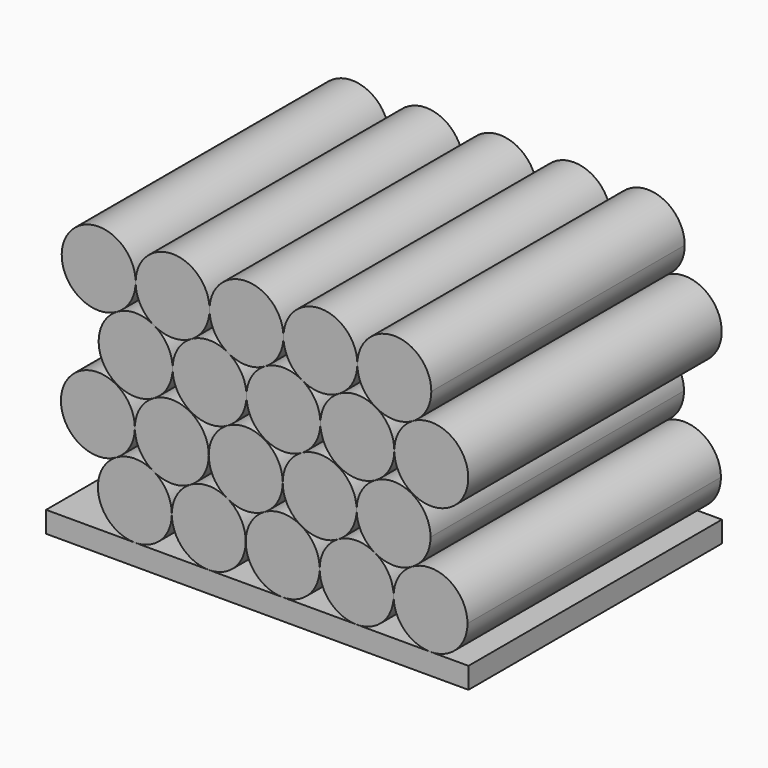
from build123d import *

# Parameters (mm, degrees)
F1_DEPTH = 76.2


# Not quite as in the source:
# - a feature names something its author has since deleted; it is built from what else it names


with BuildPart() as f1:
    # F0 (on Front) → F1 (new body)
    with BuildSketch(Plane.XZ):
        with BuildLine():
            ThreePointArc((-29.4477027383, -25.4555717693), (-23.1615234536, -22.851751054), (-20.5577027383, -16.5655717693))
            ThreePointArc((-20.5577027383, -16.5655717693), (-21.7487368667, -12.1205718246), (-25.0027026277, -8.8666059935))
            ThreePointArc((-25.0027026277, -8.8666059935), (-29.4477026803, -7.6755717693), (-33.8927027485, -8.8666059355))
            ThreePointArc((-33.8927027485, -8.8666059355), (-38.0347833325, -18.8664730859), (-29.4477027383, -25.4555717693))
        make_face()
    extrude(amount=F1_DEPTH)


with BuildPart() as f1b:
    # F0 (on Front) → F1, piece 2 (new body)
    with BuildSketch(Plane.XZ):
        with BuildLine():
            ThreePointArc((-16.1127027426, -8.8666059321), (-19.3666685792, -12.1205717714), (-20.5577027383, -16.5655717693))
            ThreePointArc((-20.5577027383, -16.5655717693), (-17.9538820218, -22.8517510553), (-11.6677027346, -25.4555717693))
            ThreePointArc((-11.6677027346, -25.4555717693), (-5.3815234523, -22.8517510527), (-2.7777027383, -16.5655717693))
            ThreePointArc((-2.7777027383, -16.5655717693), (-3.9687368512, -12.1205718515), (-7.2227025739, -8.8666060246))
            ThreePointArc((-7.2227025739, -8.8666060246), (-11.6677026458, -7.6755717693), (-16.1127027426, -8.8666059321))
        make_face()
    extrude(amount=F1_DEPTH)


with BuildPart() as f1c:
    # F0 (on Front) → F1, piece 3 (new body)
    with BuildSketch(Plane.XZ):
        with BuildLine():
            ThreePointArc((-29.4477027383, -1.16764009), (-28.256668546, -5.6126401453), (-25.0027026277, -8.8666059935))
            ThreePointArc((-25.0027026277, -8.8666059935), (-20.5577026769, -10.05764009), (-16.1127027426, -8.8666059321))
            ThreePointArc((-16.1127027426, -8.8666059321), (-12.8587368999, -5.6126400921), (-11.6677027383, -1.16764009))
            ThreePointArc((-11.6677027383, -1.16764009), (-16.0669411864, 6.5047233453), (-24.9107085164, 6.5837108049))
            ThreePointArc((-24.9107085164, 6.5837108049), (-28.2300661736, 3.323121462), (-29.4477027383, -1.16764009))
        make_face()
    extrude(amount=F1_DEPTH)


with BuildPart() as f1d:
    # F0 (on Front) → F1, piece 4 (new body)
    with BuildSketch(Plane.XZ):
        Polygon((-11.6677027346, -25.4555717693), (-29.4477027383, -25.4555717693), (-50.8, -25.4555717693), (-50.8, -30.5355717693), (50.8, -30.5355717693), (50.8, -25.4555717693), (41.6722971921, -25.4555717693), (23.8922972402, -25.4555717693), (6.1122972617, -25.4555717693), align=None)
    extrude(amount=F1_DEPTH)


with BuildPart() as f1e:
    # F0 (on Front) → F1, piece 5 (new body)
    with BuildSketch(Plane.XZ):
        with BuildLine():
            ThreePointArc((-29.4477027383, -1.16764009), (-46.036668575, 3.2773599151), (-33.8927027485, -8.8666059355))
            ThreePointArc((-33.8927027485, -8.8666059355), (-30.6387369016, -5.6126400951), (-29.4477027383, -1.16764009))
        make_face()
    extrude(amount=F1_DEPTH)


with BuildPart() as f1f:
    # F0 (on Front) → F1, piece 6 (new body)
    with BuildSketch(Plane.XZ):
        with BuildLine():
            ThreePointArc((-11.6677027383, -1.16764009), (-10.4766685305, -5.6126401722), (-7.2227025739, -8.8666060246))
            ThreePointArc((-7.2227025739, -8.8666060246), (-2.7777025673, -10.05764009), (1.6672973934, -8.8666058536))
            ThreePointArc((1.6672973934, -8.8666058536), (4.9212631394, -5.6126400241), (6.1122972617, -1.16764009))
            ThreePointArc((6.1122972617, -1.16764009), (1.7130586982, 6.5047234129), (-7.1307087496, 6.583710674))
            ThreePointArc((-7.1307087496, 6.583710674), (-10.4500662412, 3.3231213466), (-11.6677027383, -1.16764009))
        make_face()
    extrude(amount=F1_DEPTH)


with BuildPart() as f1g:
    # F0 (on Front) → F1, piece 7 (new body)
    with BuildSketch(Plane.XZ):
        with BuildLine():
            ThreePointArc((1.6672973934, -8.8666058536), (-1.5866685399, -12.1205717034), (-2.7777027383, -16.5655717693))
            ThreePointArc((-2.7777027383, -16.5655717693), (-0.1738820231, -22.851751054), (6.1122972617, -25.4555717693))
            ThreePointArc((6.1122972617, -25.4555717693), (12.3984765464, -22.851751054), (15.0022972617, -16.5655717693))
            ThreePointArc((15.0022972617, -16.5655717693), (13.8112631619, -12.1205718742), (10.5572974715, -8.8666060508))
            ThreePointArc((10.5572974715, -8.8666060508), (6.1122974589, -7.6755717693), (1.6672973934, -8.8666058536))
        make_face()
    extrude(amount=F1_DEPTH)


with BuildPart() as f1h:
    # F0 (on Front) → F1, piece 8 (new body)
    with BuildSketch(Plane.XZ):
        with BuildLine():
            ThreePointArc((-33.7087146145, 22.0340273618), (-36.9890099597, 9.935980421), (-24.9107085164, 6.5837108049))
            ThreePointArc((-24.9107085164, 6.5837108049), (-21.5913511801, 9.8443001178), (-20.3737147463, 14.3350614461))
            ThreePointArc((-20.3737147463, 14.3350614461), (-21.564748866, 18.7800613757), (-24.8187146054, 22.0340272044))
            ThreePointArc((-24.8187146054, 22.0340272044), (-29.2637145889, 23.2250614461), (-33.7087146145, 22.0340273618))
        make_face()
    extrude(amount=F1_DEPTH)


with BuildPart() as f1i:
    # F0 (on Front) → F1, piece 9 (new body)
    with BuildSketch(Plane.XZ):
        with BuildLine():
            ThreePointArc((-20.3737147463, 14.3350614461), (-15.97447619, 6.6626979475), (-7.1307087496, 6.583710674))
            ThreePointArc((-7.1307087496, 6.583710674), (-3.8113512476, 9.8443000024), (-2.5937147463, 14.3350614461))
            ThreePointArc((-2.5937147463, 14.3350614461), (-3.7847488029, 18.7800612665), (-7.0387143871, 22.0340270784))
            ThreePointArc((-7.0387143871, 22.0340270784), (-11.483714467, 23.2250614461), (-15.9287146218, 22.0340273576))
            ThreePointArc((-15.9287146218, 22.0340273576), (-19.18268055, 18.7800615083), (-20.3737147463, 14.3350614461))
        make_face()
    extrude(amount=F1_DEPTH)


with BuildPart() as f1j:
    # F0 (on Front) → F1, piece 10 (new body)
    with BuildSketch(Plane.XZ):
        with BuildLine():
            ThreePointArc((19.4472973755, -8.8666058639), (16.1933314549, -12.1205717124), (15.0022972617, -16.5655717693))
            ThreePointArc((15.0022972617, -16.5655717693), (17.6061179693, -22.8517510464), (23.8922972402, -25.4555717693))
            ThreePointArc((23.8922972402, -25.4555717693), (30.1784765388, -22.8517510616), (32.7822972617, -16.5655717693))
            ThreePointArc((32.7822972617, -16.5655717693), (31.5912630633, -12.1205717034), (28.3372971299, -8.8666058536))
            ThreePointArc((28.3372971299, -8.8666058536), (23.8922972513, -7.6755717693), (19.4472973755, -8.8666058639))
        make_face()
    extrude(amount=F1_DEPTH)


with BuildPart() as f1k:
    # F0 (on Front) → F1, piece 11 (new body)
    with BuildSketch(Plane.XZ):
        with BuildLine():
            ThreePointArc((-29.2637147463, 29.7329931254), (-45.852680624, 34.1779930595), (-33.7087146145, 22.0340273618))
            ThreePointArc((-33.7087146145, 22.0340273618), (-30.4547488686, 25.2879931913), (-29.2637147463, 29.7329931254))
        make_face()
    extrude(amount=F1_DEPTH)


with BuildPart() as f1l:
    # F0 (on Front) → F1, piece 12 (new body)
    with BuildSketch(Plane.XZ):
        with BuildLine():
            ThreePointArc((6.1122972617, -1.16764009), (7.3033314826, -5.6126401949), (10.5572974715, -8.8666060508))
            ThreePointArc((10.5572974715, -8.8666060508), (15.0022974485, -10.05764009), (19.4472973755, -8.8666058639))
            ThreePointArc((19.4472973755, -8.8666058639), (22.7012631342, -5.6126400331), (23.8922972617, -1.16764009))
            ThreePointArc((23.8922972617, -1.16764009), (19.4930587398, 6.5047233886), (10.6492913344, 6.5837107211))
            ThreePointArc((10.6492913344, 6.5837107211), (7.3299337831, 3.3231213881), (6.1122972617, -1.16764009))
        make_face()
    extrude(amount=F1_DEPTH)


with BuildPart() as f1m:
    # F0 (on Front) → F1, piece 13 (new body)
    with BuildSketch(Plane.XZ):
        with BuildLine():
            ThreePointArc((1.8512849925, 22.0340271349), (-1.4026806613, 18.7800613155), (-2.5937147463, 14.3350614461))
            ThreePointArc((-2.5937147463, 14.3350614461), (1.8055238515, 6.6626979231), (10.6492913344, 6.5837107211))
            ThreePointArc((10.6492913344, 6.5837107211), (13.9686487767, 9.8443000439), (15.1862852537, 14.3350614461))
            ThreePointArc((15.1862852537, 14.3350614461), (13.9952512129, 18.7800612391), (10.7412856677, 22.0340270467))
            ThreePointArc((10.7412856677, 22.0340270467), (6.2962853419, 23.2250614461), (1.8512849925, 22.0340271349))
        make_face()
    extrude(amount=F1_DEPTH)


with BuildPart() as f1n:
    # F0 (on Front) → F1, piece 14 (new body)
    with BuildSketch(Plane.XZ):
        with BuildLine():
            ThreePointArc((37.2272973436, -8.8666058823), (33.9733314457, -12.1205717283), (32.7822972617, -16.5655717693))
            ThreePointArc((32.7822972617, -16.5655717693), (35.3861179524, -22.8517510294), (41.6722971921, -25.4555717693))
            ThreePointArc((41.6722971921, -25.4555717693), (47.9584765218, -22.8517510786), (50.5622972617, -16.5655717693))
            ThreePointArc((50.5622972617, -16.5655717693), (46.1172973026, -8.8666059533), (37.2272973436, -8.8666058823))
        make_face()
    extrude(amount=F1_DEPTH)


with BuildPart() as f1o:
    # F0 (on Front) → F1, piece 15 (new body)
    with BuildSketch(Plane.XZ):
        with BuildLine():
            ThreePointArc((-29.2637147463, 29.7329931254), (-28.0726805453, 25.2879930549), (-24.8187146054, 22.0340272044))
            ThreePointArc((-24.8187146054, 22.0340272044), (-20.3737145931, 20.8429931254), (-15.9287146218, 22.0340273576))
            ThreePointArc((-15.9287146218, 22.0340273576), (-12.6747488707, 25.2879931876), (-11.4837147463, 29.7329931254))
            ThreePointArc((-11.4837147463, 29.7329931254), (-20.3737147463, 38.6229931254), (-29.2637147463, 29.7329931254))
        make_face()
    extrude(amount=F1_DEPTH)


with BuildPart() as f1p:
    # F0 (on Front) → F1, piece 16 (new body)
    with BuildSketch(Plane.XZ):
        with BuildLine():
            ThreePointArc((-11.4837147463, 29.7329931254), (-10.2926804822, 25.2879929458), (-7.0387143871, 22.0340270784))
            ThreePointArc((-7.0387143871, 22.0340270784), (-2.5937146897, 20.8429931254), (1.8512849925, 22.0340271349))
            ThreePointArc((1.8512849925, 22.0340271349), (5.1052510179, 25.2879929948), (6.2962852537, 29.7329931254))
            ThreePointArc((6.2962852537, 29.7329931254), (-2.5937147463, 38.6229931254), (-11.4837147463, 29.7329931254))
        make_face()
    extrude(amount=F1_DEPTH)


with BuildPart() as f1q:
    # F0 (on Front) → F1, piece 17 (new body)
    with BuildSketch(Plane.XZ):
        with BuildLine():
            ThreePointArc((23.8922972617, -1.16764009), (25.083331384, -5.6126400241), (28.3372971299, -8.8666058536))
            ThreePointArc((28.3372971299, -8.8666058536), (32.7822972329, -10.05764009), (37.2272973436, -8.8666058823))
            ThreePointArc((37.2272973436, -8.8666058823), (40.481263125, -5.612640049), (41.6722972617, -1.16764009))
            ThreePointArc((41.6722972617, -1.16764009), (37.2730586761, 6.5047234258), (28.4292912057, 6.5837106489))
            ThreePointArc((28.4292912057, 6.5837106489), (25.1099337459, 3.3231213244), (23.8922972617, -1.16764009))
        make_face()
    extrude(amount=F1_DEPTH)


with BuildPart() as f1r:
    # F0 (on Front) → F1, piece 18 (new body)
    with BuildSketch(Plane.XZ):
        with BuildLine():
            ThreePointArc((19.6312850473, 22.0340271665), (16.3773193545, 18.7800613429), (15.1862852537, 14.3350614461))
            ThreePointArc((15.1862852537, 14.3350614461), (19.5855237879, 6.6626979604), (28.4292912057, 6.5837106489))
            ThreePointArc((28.4292912057, 6.5837106489), (31.7486487394, 9.8442999802), (32.9662852537, 14.3350614461))
            ThreePointArc((32.9662852537, 14.3350614461), (31.7752512108, 18.7800612428), (28.5212856604, 22.034027051))
            ThreePointArc((28.5212856604, 22.034027051), (24.0762853693, 23.2250614461), (19.6312850473, 22.0340271665))
        make_face()
    extrude(amount=F1_DEPTH)


with BuildPart() as f1s:
    # F0 (on Front) → F1, piece 19 (new body)
    with BuildSketch(Plane.XZ):
        with BuildLine():
            ThreePointArc((6.2962852537, 29.7329931254), (7.4873195336, 25.2879929184), (10.7412856677, 22.0340270467))
            ThreePointArc((10.7412856677, 22.0340270467), (15.1862853735, 20.8429931254), (19.6312850473, 22.0340271665))
            ThreePointArc((19.6312850473, 22.0340271665), (22.8852510338, 25.2879930222), (24.0762852537, 29.7329931254))
            ThreePointArc((24.0762852537, 29.7329931254), (15.1862852537, 38.6229931254), (6.2962852537, 29.7329931254))
        make_face()
    extrude(amount=F1_DEPTH)


with BuildPart() as f1t:
    # F0 (on Front) → F1, piece 20 (new body)
    with BuildSketch(Plane.XZ):
        with BuildLine():
            ThreePointArc((41.8562852537, 29.7329931254), (32.9662852537, 38.6229931254), (24.0762852537, 29.7329931254))
            ThreePointArc((24.0762852537, 29.7329931254), (25.2673195315, 25.2879929221), (28.5212856604, 22.034027051))
            ThreePointArc((28.5212856604, 22.034027051), (32.9662856111, 20.8429931254), (37.4112854661, 22.0340274083))
            ThreePointArc((37.4112854661, 22.0340274083), (40.6652511547, 25.2879932316), (41.8562852537, 29.7329931254))
        make_face()
    extrude(amount=F1_DEPTH)


with BuildPart() as f1u:
    # F0 (on Front) → F1, piece 21 (new body)
    with BuildSketch(Plane.XZ):
        with BuildLine():
            ThreePointArc((37.4112854661, 22.0340274083), (34.1573194754, 18.7800615523), (32.9662852537, 14.3350614461))
            ThreePointArc((32.9662852537, 14.3350614461), (41.8562852537, 5.4450614461), (50.7462852537, 14.3350614461))
            ThreePointArc((50.7462852537, 14.3350614461), (46.3012853599, 22.0340272244), (37.4112854661, 22.0340274083))
        make_face()
    extrude(amount=F1_DEPTH)


solid = Compound([f1.part, f1b.part, f1c.part, f1d.part, f1e.part, f1f.part, f1g.part, f1h.part, f1i.part, f1j.part, f1k.part, f1l.part, f1m.part, f1n.part, f1o.part, f1p.part, f1q.part, f1r.part, f1s.part, f1t.part, f1u.part])
